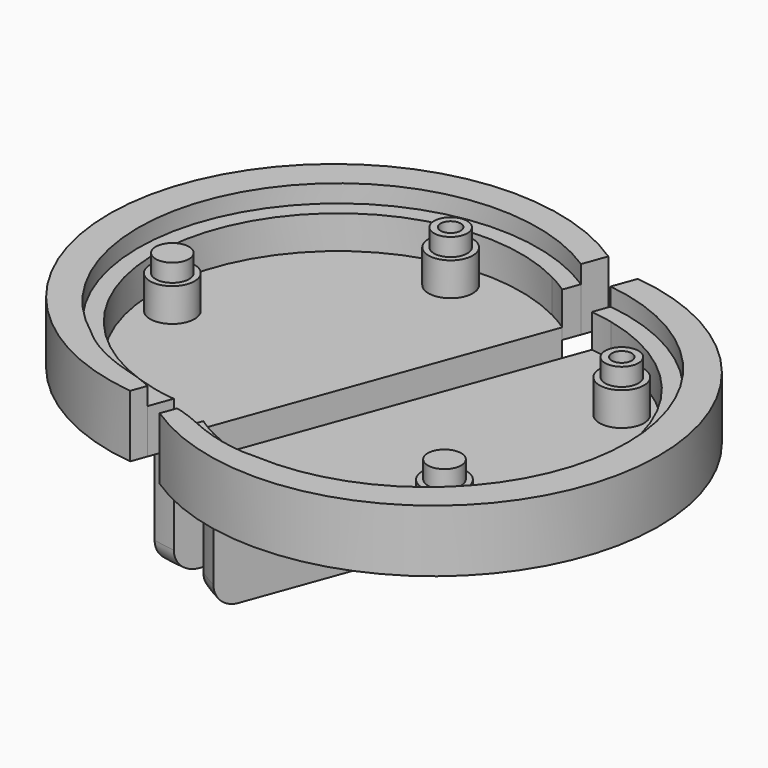
from build123d import *

# Parameters (mm, degrees)
F3_R     = 2
F4_DEPTH = 1
F3_R_2   = 1.5
F5_DEPTH = 4
F3_R_3   = 0.9
F6_DEPTH = 5.6
F7_DEPTH = 10
F8_R     = 2


# Not quite as in the source:
# - a feature names something its author has since deleted; it is built from what else it names


with BuildPart() as f4:
    # F3 (on Top) → F4 (new body)
    with BuildSketch(Plane.XY):
        with BuildLine():
            ThreePointArc((24.4428970275, -14.671741632), (47.4729130652, -5.6368234206), (35.645763749, 16.0917274937))
            Line((35.645763749, 16.0917274937), (24.4428970275, -14.671741632))
        make_face()
        with Locations((41.5076157406, -9.9849013437)):
            Circle(F3_R, mode=Mode.SUBTRACT)
        with Locations((41.5070735985, 9.9851724147)):
            Circle(F3_R, mode=Mode.SUBTRACT)
        with BuildLine():
            ThreePointArc((35.645763749, 16.0917274937), (34.656487532, 16.286160575), (33.6571820844, 16.4198029295))
            Line((33.6571820844, 16.4198029295), (22.7090189654, -13.6442410753))
            ThreePointArc((22.7090189654, -13.6442410753), (23.5602527059, -14.1844935862), (24.4428970275, -14.671741632))
            Line((24.4428970275, -14.671741632), (35.645763749, 16.0917274937))
        make_face()
    extrude(amount=F4_DEPTH)

    # F3 (on Top) → F5 (join)
    with BuildSketch(Plane.XY):
        with BuildLine():
            Line((29.7526022679, -17.9595595539), (30.8971311949, -17.9595595539))
            ThreePointArc((30.8971311949, -17.9595595539), (49.8956420488, -1.6368218512), (34.185866977, 17.871590385))
            Line((34.185866977, 17.871590385), (33.6571820844, 16.4198029295))
            ThreePointArc((33.6571820844, 16.4198029295), (34.656487532, 16.286160575), (35.645763749, 16.0917274937))
            ThreePointArc((35.645763749, 16.0917274937), (47.4729130652, -5.6368234206), (24.4428970275, -14.671741632))
            ThreePointArc((24.4428970275, -14.671741632), (23.5602527059, -14.1844935862), (22.7090189654, -13.6442410753))
            Line((22.7090189654, -13.6442410753), (21.9645680543, -15.6885296658))
            Line((21.9645680543, -15.6885296658), (22.4073752761, -15.7830882818))
            Line((22.4073752761, -15.7830882818), (23.4502572566, -16.1368325353))
            Line((23.4502572566, -16.1368325353), (25.4884753376, -17.0060619712))
            Line((25.4884753376, -17.0060619712), (26.5388786793, -17.3585340381))
            Line((26.5388786793, -17.3585340381), (27.5754574686, -17.6364984363))
            Line((27.5754574686, -17.6364984363), (28.6447145045, -17.8397707641))
            Line((28.6447145045, -17.8397707641), (29.7526022679, -17.9595595539))
        make_face()
        with Locations((41.5076157406, -9.9849013437)):
            Circle(F3_R)
        with Locations((41.5076157406, -9.9849013437)):
            Circle(F3_R_2, mode=Mode.SUBTRACT)
        with Locations((41.5070735985, 9.9851724147)):
            Circle(F3_R)
        with Locations((41.5070735985, 9.9851724147)):
            Circle(F3_R_2, mode=Mode.SUBTRACT)
    extrude(amount=F5_DEPTH)

    # F3 (on Top) → F6 (join)
    with BuildSketch(Plane.XY):
        with BuildLine():
            ThreePointArc((34.185866977, 17.871590385), (49.8956420488, -1.6368218512), (30.8971311949, -17.9595595539))
            Line((30.8971311949, -17.9595595539), (29.7526022679, -17.9595595539))
            Line((29.7526022679, -17.9595595539), (28.6447145045, -17.8397707641))
            Line((28.6447145045, -17.8397707641), (27.5754574686, -17.6364984363))
            Line((27.5754574686, -17.6364984363), (26.5388786793, -17.3585340381))
            Line((26.5388786793, -17.3585340381), (25.4884753376, -17.0060619712))
            Line((25.4884753376, -17.0060619712), (23.4502572566, -16.1368325353))
            Line((23.4502572566, -16.1368325353), (22.4073752761, -15.7830882818))
            Line((22.4073752761, -15.7830882818), (21.9645680543, -15.6885296658))
            Line((21.9645680543, -15.6885296658), (21.4785924091, -17.0230360138))
            ThreePointArc((21.4785924091, -17.0230360138), (51.7265670481, -7.0799100929), (34.9557263509, 19.985651515))
            Line((34.9557263509, 19.985651515), (34.185866977, 17.871590385))
        make_face()
        with Locations((41.5076157406, -9.9849013437)):
            Circle(F3_R_2)
        with Locations((41.5070735985, 9.9851724147)):
            Circle(F3_R_2)
        with Locations((41.5070735985, 9.9851724147)):
            Circle(F3_R_3, mode=Mode.SUBTRACT)
    extrude(amount=F6_DEPTH)

    # F3 (on Top) → F7 (join)
    with BuildSketch(Plane.XY):
        with BuildLine():
            ThreePointArc((35.645763749, 16.0917274937), (34.656487532, 16.286160575), (33.6571820844, 16.4198029295))
            Line((33.6571820844, 16.4198029295), (22.7090189654, -13.6442410753))
            ThreePointArc((22.7090189654, -13.6442410753), (23.5602527059, -14.1844935862), (24.4428970275, -14.671741632))
            Line((24.4428970275, -14.671741632), (35.645763749, 16.0917274937))
        make_face()
    extrude(amount=-F7_DEPTH)

    # F8
    f8_edges = [f4.edges().sort_by_distance(p)[0] for p in [
        (23.560253, -14.184494, -10),
        (34.656488, 16.286161, -10),
    ]]
    fillet(f8_edges, radius=F8_R)


with BuildPart() as f10_1:
    # F10: instance of F4
    add(f4.part.mirror(Plane(origin=(26.3392995557, 2.1695369703, -3.8368049067), x_dir=(-0.3421787181, -0.9396348891, 0), z_dir=(-0.9396348891, 0.3421787181, 0))))


solid = Compound([f4.part, f10_1.part])
